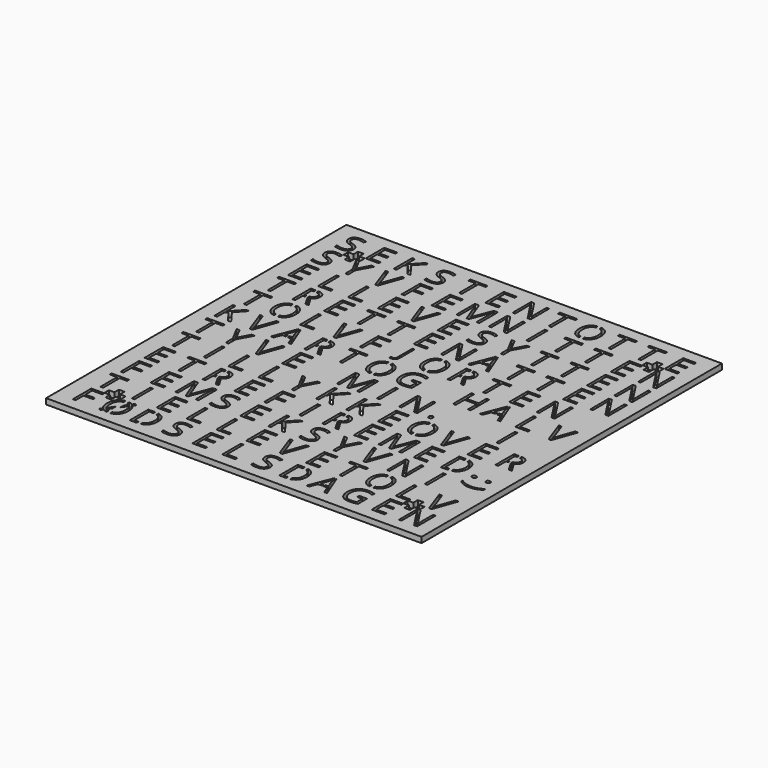
from build123d import *

# Parameters (mm, degrees)
F0_W            = 195
F0_H            = 195
F1_DEPTH        = 3
F2_W            = 3
F2_H            = 3
F3_DEPTH        = 3.001
F5_TEXT_SIZE    = 17.3611111111
F28_DEPTH       = 3.001
F6_TEXT_SIZE    = 17.3611111111
F29_DEPTH       = 3.0010001
F7_TEXT_SIZE    = 17.3611111111
F30_DEPTH       = 3.0010001
F8_TEXT_SIZE    = 17.3611111111
F31_DEPTH       = 3.0010001
F9_TEXT_SIZE    = 17.3611111111
F32_DEPTH       = 3.0010001
F10_TEXT_SIZE   = 17.3611111111
F33_DEPTH       = 3.0010001
F11_TEXT_SIZE   = 17.3611111111
F34_DEPTH       = 3.0010001
F12_TEXT_SIZE   = 17.3611111111
F12_TEXT_SIZE_2 = 13.8888888889
F35_DEPTH       = 3.0010001
F13_TEXT_SIZE   = 17.3611111111
F36_DEPTH       = 3.0010001
F14_TEXT_SIZE   = 17.3611111111
F37_DEPTH       = 3.0010001
F15_TEXT_SIZE   = 17.3611111111
F38_DEPTH       = 3.0010001
F16_TEXT_SIZE   = 17.3611111111
F17_TEXT_SIZE   = 17.3611111111
F18_TEXT_SIZE   = 17.3611111111
F39_DEPTH       = 3.0010001
F19_TEXT_SIZE   = 17.3611111111
F40_DEPTH       = 3.0010001
F20_TEXT_SIZE   = 17.3611111111
F41_DEPTH       = 3.0010001
F21_TEXT_SIZE   = 17.3611111111
F42_DEPTH       = 3.0010001
F24_TEXT_SIZE   = 17.3611111111
F22_TEXT_SIZE   = 17.3611111111
F23_TEXT_SIZE   = 17.3611111111
F23_TEXT_SIZE_2 = 13.8888888889
F43_DEPTH       = 3.0010001
F25_TEXT_SIZE   = 17.3611111111
F44_DEPTH       = 3.0010001
F26_TEXT_SIZE   = 17.3611111111
F45_DEPTH       = 3.0010001
F27_TEXT_SIZE   = 17.3611111111
F46_DEPTH       = 25
F47_DEPTH       = 3
F48_DEPTH       = 3
F49_DEPTH       = 3
F50_DEPTH       = 3


# Not quite as in the source:
# - Text() gives the source's letters only with a copy of the font that has no kerning and outlines rounded to 1/6400 em; it was checked with that copy


with BuildPart() as f1:
    # F0 (on Top) → F1 (new body)
    with BuildSketch(Plane.XY):
        Rectangle(F0_W, F0_H)
    extrude(amount=F1_DEPTH)

    # F2 (on face) → F3 (cut, through all)
    with BuildSketch(Plane.XY.offset(3)):
        with Locations((-83, 80)):
            Rectangle(F2_W, F2_H)
        with Locations((-80, 80)):
            Rectangle(F2_W, F2_H)
        with Locations((-80, 83)):
            Rectangle(F2_W, F2_H)
        with Locations((-77, 80)):
            Rectangle(F2_W, F2_H)
        with Locations((-80, 77)):
            Rectangle(F2_W, F2_H)
        with Locations((77, 80)):
            Rectangle(F2_W, F2_H)
        with Locations((80, 83)):
            Rectangle(F2_W, F2_H)
        with Locations((80, 77)):
            Rectangle(F2_W, F2_H)
        with Locations((83, 80)):
            Rectangle(F2_W, F2_H)
        with Locations((80, 80)):
            Rectangle(F2_W, F2_H)
        with Locations((80, -80)):
            Rectangle(F2_W, F2_H)
        with Locations((-80, -83)):
            Rectangle(F2_W, F2_H)
        with Locations((80, -83)):
            Rectangle(F2_W, F2_H)
        with Locations((77, -80)):
            Rectangle(F2_W, F2_H)
        with Locations((-80, -80)):
            Rectangle(F2_W, F2_H)
        with Locations((-80, -77)):
            Rectangle(F2_W, F2_H)
        with Locations((-83, -80)):
            Rectangle(F2_W, F2_H)
        with Locations((-77, -80)):
            Rectangle(F2_W, F2_H)
        with Locations((83, -80)):
            Rectangle(F2_W, F2_H)
        with Locations((80, -77)):
            Rectangle(F2_W, F2_H)
    extrude(amount=-F3_DEPTH, mode=Mode.SUBTRACT)

    # F5 (on face) → F28 (cut, through all)
    with BuildSketch(Plane.XY.offset(3)):
        with BuildLine():
            add(Edge.make_bspline(
                [(41, 94.2741594654), (42.9624487495, 94.006635936), (44.1680230035, 92.6440972222)],
                knots=[0.1963419657, 0.1963419657, 0.1963419657, 1, 1, 1], degree=2))
            Line((41, 94.2741594654), (41, 92.9625807227))
            add(Edge.make_bspline(
                [(43.0938042535, 91.7584092882), (42.3205692357, 92.7129338633), (41, 92.9625807227)],
                knots=[0, 0, 0, 0.738459474, 0.738459474, 0.738459474], degree=2))
            add(Edge.make_bspline(
                [(44.1408962674, 87.9647352431), (44.1408962674, 90.4658203125), (43.0938042535, 91.7584092882)],
                knots=[0, 0, 0, 1, 1, 1], degree=2))
            add(Edge.make_bspline(
                [(43.0897352431, 84.1398654514), (44.1408962674, 85.4365234375), (44.1408962674, 87.9647352431)],
                knots=[0, 0, 0, 1, 1, 1], degree=2))
            add(Edge.make_bspline(
                [(41, 82.9342437314), (42.3170989399, 83.1867811858), (43.0897352431, 84.1398654514)],
                knots=[0.2649686534, 0.2649686534, 0.2649686534, 1, 1, 1], degree=2))
            Line((41, 82.9342437314), (41, 81.6467767811))
            add(Edge.make_bspline(
                [(44.1625976562, 83.2840169271), (42.9570173112, 81.9187786444), (41, 81.6467767811)],
                knots=[0, 0, 0, 0.8007660152, 0.8007660152, 0.8007660152], degree=2))
            add(Edge.make_bspline(
                [(45.6681315104, 87.9647352431), (45.6681315104, 84.9889322917), (44.1625976562, 83.2840169271)],
                knots=[0, 0, 0, 1, 1, 1], degree=2))
            add(Edge.make_bspline(
                [(44.1680230035, 92.6440972222), (45.6681315104, 90.9486762153), (45.6681315104, 87.9647352431)],
                knots=[0, 0, 0, 1, 1, 1], degree=2))
        make_face()
        with BuildLine():
            Line((39, 92.9644818436), (39, 94.2796444382))
            add(Edge.make_bspline(
                [(35.758734809, 92.6739366319), (36.9678295875, 94.0237260755), (39, 94.2796444382)],
                knots=[0, 0, 0, 0.8104012711, 0.8104012711, 0.8104012711], degree=2))
            add(Edge.make_bspline(
                [(34.2667643229, 87.9810112847), (34.2667643229, 91.0083550347), (35.758734809, 92.6739366319)],
                knots=[0, 0, 0, 1, 1, 1], degree=2))
            add(Edge.make_bspline(
                [(35.7546657986, 83.2541775174), (34.2667643229, 84.9292534722), (34.2667643229, 87.9810112847)],
                knots=[0, 0, 0, 1, 1, 1], degree=2))
            add(Edge.make_bspline(
                [(39, 81.6376356301), (36.9644286676, 81.8922293467), (35.7546657986, 83.2541775174)],
                knots=[0.186933484, 0.186933484, 0.186933484, 1, 1, 1], degree=2))
            Line((39, 81.6376356301), (39, 82.9280543594))
            add(Edge.make_bspline(
                [(36.8641493056, 84.1452907986), (37.6631428834, 83.1755893641), (39, 82.9280543594)],
                knots=[0, 0, 0, 0.7447307017, 0.7447307017, 0.7447307017], degree=2))
            add(Edge.make_bspline(
                [(35.7912868924, 87.9647352431), (35.7912868924, 85.4473741319), (36.8641493056, 84.1452907986)],
                knots=[0, 0, 0, 1, 1, 1], degree=2))
            add(Edge.make_bspline(
                [(36.8641493056, 91.7489149306), (35.7912868924, 90.4468315972), (35.7912868924, 87.9647352431)],
                knots=[0, 0, 0, 1, 1, 1], degree=2))
            add(Edge.make_bspline(
                [(39, 92.9644818436), (37.6604615605, 92.7153621678), (36.8641493056, 91.7489149306)],
                knots=[0.2577685218, 0.2577685218, 0.2577685218, 1, 1, 1], degree=2))
        make_face()
        with Locations((50.7157118056, 81.75)):
            Text('T', F5_TEXT_SIZE, font='Open Sans', text_align=(TextAlign.LEFT, TextAlign.BOTTOM))
        with Locations((18.7157118056, 81.75)):
            Text('T', F5_TEXT_SIZE, font='Open Sans', text_align=(TextAlign.LEFT, TextAlign.BOTTOM))
        with Locations((1.7445746528, 81.75)):
            Text('N', F5_TEXT_SIZE, font='Open Sans', text_align=(TextAlign.LEFT, TextAlign.BOTTOM))
        with Locations((-12.8692491319, 81.75)):
            Text('E', F5_TEXT_SIZE, font='Open Sans', text_align=(TextAlign.LEFT, TextAlign.BOTTOM))
        with Locations((-29.2842881944, 81.75)):
            Text('T', F5_TEXT_SIZE, font='Open Sans', text_align=(TextAlign.LEFT, TextAlign.BOTTOM))
        with Locations((-44.9112955729, 81.75)):
            Text('S', F5_TEXT_SIZE, font='Open Sans', text_align=(TextAlign.LEFT, TextAlign.BOTTOM))
        with Locations((-61.8905707465, 81.75)):
            Text('K', F5_TEXT_SIZE, font='Open Sans', text_align=(TextAlign.LEFT, TextAlign.BOTTOM))
        with Locations((-76.8692491319, 81.75)):
            Text('E', F5_TEXT_SIZE, font='Open Sans', text_align=(TextAlign.LEFT, TextAlign.BOTTOM))
        with Locations((-92.9112955729, 81.75)):
            Text('S', F5_TEXT_SIZE, font='Open Sans', text_align=(TextAlign.LEFT, TextAlign.BOTTOM))
    extrude(amount=-F28_DEPTH, mode=Mode.SUBTRACT)

    # F6 (on face) → F29 (cut, through all)
    with BuildSketch(Plane.XY.offset(3)):
        with Locations((66.7157118056, 81.75)):
            Text('T', F6_TEXT_SIZE, font='Open Sans', text_align=(TextAlign.LEFT, TextAlign.BOTTOM))
        with Locations((83.1307508681, 81.75)):
            Text('E', F6_TEXT_SIZE, font='Open Sans', text_align=(TextAlign.LEFT, TextAlign.BOTTOM))
    extrude(amount=-F29_DEPTH, mode=Mode.SUBTRACT)

    # F7 (on face) → F30 (cut, through all)
    with BuildSketch(Plane.XY.offset(3)):
        with Locations((-92.9112955729, 65.75)):
            Text('S', F7_TEXT_SIZE, font='Open Sans', text_align=(TextAlign.LEFT, TextAlign.BOTTOM))
        with Locations((-77.4239908854, 65.75)):
            Text('Y', F7_TEXT_SIZE, font='Open Sans', text_align=(TextAlign.LEFT, TextAlign.BOTTOM))
        with Locations((-61.7291666667, 65.75)):
            Text('V', F7_TEXT_SIZE, font='Open Sans', text_align=(TextAlign.LEFT, TextAlign.BOTTOM))
        with Locations((-44.8692491319, 65.75)):
            Text('F', F7_TEXT_SIZE, font='Open Sans', text_align=(TextAlign.LEFT, TextAlign.BOTTOM))
        with Locations((-28.8692491319, 65.75)):
            Text('E', F7_TEXT_SIZE, font='Open Sans', text_align=(TextAlign.LEFT, TextAlign.BOTTOM))
        with Locations((-15.5520833333, 65.75)):
            Text('M', F7_TEXT_SIZE, font='Open Sans', text_align=(TextAlign.LEFT, TextAlign.BOTTOM))
        with Locations((1.7445746528, 65.75)):
            Text('N', F7_TEXT_SIZE, font='Open Sans', text_align=(TextAlign.LEFT, TextAlign.BOTTOM))
        with Locations((21.8651258681, 65.75)):
            Text('I', F7_TEXT_SIZE, font='Open Sans', text_align=(TextAlign.LEFT, TextAlign.BOTTOM))
        with Locations((34.7157118056, 65.75)):
            Text('T', F7_TEXT_SIZE, font='Open Sans', text_align=(TextAlign.LEFT, TextAlign.BOTTOM))
        with Locations((50.7157118056, 65.75)):
            Text('T', F7_TEXT_SIZE, font='Open Sans', text_align=(TextAlign.LEFT, TextAlign.BOTTOM))
        with Locations((67.1307508681, 65.75)):
            Text('E', F7_TEXT_SIZE, font='Open Sans', text_align=(TextAlign.LEFT, TextAlign.BOTTOM))
        with Locations((81.7445746528, 65.75)):
            Text('N', F7_TEXT_SIZE, font='Open Sans', text_align=(TextAlign.LEFT, TextAlign.BOTTOM))
    extrude(amount=-F30_DEPTH, mode=Mode.SUBTRACT)

    # F8 (on face) → F31 (cut, through all)
    with BuildSketch(Plane.XY.offset(3)):
        with Locations((-92.8692491319, 49.75)):
            Text('E', F8_TEXT_SIZE, font='Open Sans', text_align=(TextAlign.LEFT, TextAlign.BOTTOM))
        with Locations((-76.8692491319, 49.75)):
            Text('L', F8_TEXT_SIZE, font='Open Sans', text_align=(TextAlign.LEFT, TextAlign.BOTTOM))
        with Locations((-60.8692491319, 49.75)):
            Text('L', F8_TEXT_SIZE, font='Open Sans', text_align=(TextAlign.LEFT, TextAlign.BOTTOM))
        with Locations((-44.8692491319, 49.75)):
            Text('E', F8_TEXT_SIZE, font='Open Sans', text_align=(TextAlign.LEFT, TextAlign.BOTTOM))
        with Locations((-29.7291666667, 49.75)):
            Text('V', F8_TEXT_SIZE, font='Open Sans', text_align=(TextAlign.LEFT, TextAlign.BOTTOM))
        with Locations((-12.8692491319, 49.75)):
            Text('E', F8_TEXT_SIZE, font='Open Sans', text_align=(TextAlign.LEFT, TextAlign.BOTTOM))
    extrude(amount=-F31_DEPTH, mode=Mode.SUBTRACT)

    # F9 (on face) → F32 (cut, through all)
    with BuildSketch(Plane.XY.offset(3)):
        with Locations((3.0887044271, 49.75)):
            Text('S', F9_TEXT_SIZE, font='Open Sans', text_align=(TextAlign.LEFT, TextAlign.BOTTOM))
        with Locations((18.5760091146, 49.75)):
            Text('Y', F9_TEXT_SIZE, font='Open Sans', text_align=(TextAlign.LEFT, TextAlign.BOTTOM))
        with Locations((34.7157118056, 49.75)):
            Text('T', F9_TEXT_SIZE, font='Open Sans', text_align=(TextAlign.LEFT, TextAlign.BOTTOM))
        with Locations((50.7157118056, 49.75)):
            Text('T', F9_TEXT_SIZE, font='Open Sans', text_align=(TextAlign.LEFT, TextAlign.BOTTOM))
        with Locations((67.1307508681, 49.75)):
            Text('E', F9_TEXT_SIZE, font='Open Sans', text_align=(TextAlign.LEFT, TextAlign.BOTTOM))
        with Locations((81.7445746528, 49.75)):
            Text('N', F9_TEXT_SIZE, font='Open Sans', text_align=(TextAlign.LEFT, TextAlign.BOTTOM))
    extrude(amount=-F32_DEPTH, mode=Mode.SUBTRACT)

    # F10 (on face) → F33 (cut, through all)
    with BuildSketch(Plane.XY.offset(3)):
        with Locations((-93.2842881944, 33.75)):
            Text('T', F10_TEXT_SIZE, font='Open Sans', text_align=(TextAlign.LEFT, TextAlign.BOTTOM))
        Polygon((-74.63671875, 38.9040798611), (-73.5, 38.9040798611), (-73.5, 40.1410590278), (-74.63671875, 40.1410590278), (-74.63671875, 44.8800998264), (-73.5, 44.8800998264), (-73.5, 46.1442057292), (-76.0771484375, 46.1442057292), (-76.0771484375, 33.75), (-74.63671875, 33.75), align=None)
        with BuildLine():
            Line((-72, 40.1732229439), (-72, 38.8201979104))
            Line((-72, 38.8201979104), (-69.0486111111, 33.75))
            Line((-69.0486111111, 33.75), (-67.3450520833, 33.75))
            Line((-67.3450520833, 33.75), (-70.7114800347, 39.3191189236))
            add(Edge.make_bspline(
                [(-68.2185329861, 42.6421440972), (-68.2185329861, 40.1844618056), (-70.7114800347, 39.3191189236)],
                knots=[0, 0, 0, 1, 1, 1], degree=2))
            add(Edge.make_bspline(
                [(-69.307671441, 45.2707248264), (-68.2185329861, 44.3972439236), (-68.2185329861, 42.6421440972)],
                knots=[0, 0, 0, 1, 1, 1], degree=2))
            add(Edge.make_bspline(
                [(-72, 46.1232467952), (-70.2280998357, 46.0089015216), (-69.307671441, 45.2707248264)],
                knots=[0.1549023077, 0.1549023077, 0.1549023077, 1, 1, 1], degree=2))
            Line((-72, 46.1232467952), (-72, 44.8446421518))
            add(Edge.make_bspline(
                [(-70.4347873264, 44.3375651042), (-70.9739099068, 44.7414022431), (-72, 44.8446421518)],
                knots=[0, 0, 0, 0.7443526144, 0.7443526144, 0.7443526144], degree=2))
            add(Edge.make_bspline(
                [(-69.7105034722, 42.5661892361), (-69.7105034722, 43.7950303819), (-70.4347873264, 44.3375651042)],
                knots=[0, 0, 0, 1, 1, 1], degree=2))
            add(Edge.make_bspline(
                [(-70.4225802951, 40.7473415799), (-69.7105034722, 41.3536241319), (-69.7105034722, 42.5661892361)],
                knots=[0, 0, 0, 1, 1, 1], degree=2))
            add(Edge.make_bspline(
                [(-72, 40.1732229439), (-70.9706458163, 40.2807029362), (-70.4225802951, 40.7473415799)],
                knots=[0.2303281002, 0.2303281002, 0.2303281002, 1, 1, 1], degree=2))
        make_face()
        with Locations((-60.8692491319, 33.75)):
            Text('E', F10_TEXT_SIZE, font='Open Sans', text_align=(TextAlign.LEFT, TextAlign.BOTTOM))
        with Locations((-45.2842881944, 33.75)):
            Text('T', F10_TEXT_SIZE, font='Open Sans', text_align=(TextAlign.LEFT, TextAlign.BOTTOM))
        with Locations((-29.2842881944, 33.75)):
            Text('T', F10_TEXT_SIZE, font='Open Sans', text_align=(TextAlign.LEFT, TextAlign.BOTTOM))
        with Locations((-12.8692491319, 33.75)):
            Text('E', F10_TEXT_SIZE, font='Open Sans', text_align=(TextAlign.LEFT, TextAlign.BOTTOM))
    extrude(amount=-F33_DEPTH, mode=Mode.SUBTRACT)

    # F11 (on face) → F34 (cut, through all)
    with BuildSketch(Plane.XY.offset(3)):
        with Locations((1.7445746528, 33.75)):
            Text('N', F11_TEXT_SIZE, font='Open Sans', text_align=(TextAlign.LEFT, TextAlign.BOTTOM))
        with BuildLine():
            Line((22.9551373869, 43.0014366443), (22.9551373869, 46.1957465278))
            Line((22.9551373869, 46.1957465278), (22.8430447049, 46.1957465278))
            Line((22.8430447049, 46.1957465278), (17.9439561632, 33.75))
            Line((17.9439561632, 33.75), (19.403374566, 33.75))
            Line((19.403374566, 33.75), (20.9278971354, 37.6915147569))
            Line((20.9278971354, 37.6915147569), (22.9551373869, 37.6915147569))
            Line((22.9551373869, 37.6915147569), (22.9551373869, 38.9881727431))
            Line((22.9551373869, 38.9881727431), (21.4378797743, 38.9881727431))
            Line((21.4378797743, 38.9881727431), (22.8945855035, 42.8293185764))
            add(Edge.make_bspline(
                [(22.9551373869, 43.0014366443), (22.9254956152, 42.9160117803), (22.8945855035, 42.8293185764)],
                knots=[0.9109788783, 0.9109788783, 0.9109788783, 1, 1, 1], degree=2))
        make_face()
        with BuildLine():
            Line((24.055609809, 46.1957465278), (23.9551373869, 46.1957465278))
            Line((23.9551373869, 46.1957465278), (23.9551373869, 42.9592905556))
            add(Edge.make_bspline(
                [(24.0040690104, 42.8293185764), (23.9796652801, 42.8930525905), (23.9551373869, 42.9592905556)],
                knots=[0, 0, 0, 0.0873416616, 0.0873416616, 0.0873416616], degree=2))
            Line((24.0040690104, 42.8293185764), (25.4472113715, 38.9881727431))
            Line((25.4472113715, 38.9881727431), (23.9551373869, 38.9881727431))
            Line((23.9551373869, 38.9881727431), (23.9551373869, 37.6915147569))
            Line((23.9551373869, 37.6915147569), (25.8948025174, 37.6915147569))
            Line((25.8948025174, 37.6915147569), (27.4383138021, 33.75))
            Line((27.4383138021, 33.75), (28.9302842882, 33.75))
            Line((28.9302842882, 33.75), (24.055609809, 46.1957465278))
        make_face()
        with Locations((34.7157118056, 33.75)):
            Text('T', F11_TEXT_SIZE, font='Open Sans', text_align=(TextAlign.LEFT, TextAlign.BOTTOM))
        with Locations((50.7157118056, 33.75)):
            Text('T', F11_TEXT_SIZE, font='Open Sans', text_align=(TextAlign.LEFT, TextAlign.BOTTOM))
        with Locations((67.1307508681, 33.75)):
            Text('E', F11_TEXT_SIZE, font='Open Sans', text_align=(TextAlign.LEFT, TextAlign.BOTTOM))
        with Locations((81.7445746528, 33.75)):
            Text('N', F11_TEXT_SIZE, font='Open Sans', text_align=(TextAlign.LEFT, TextAlign.BOTTOM))
    extrude(amount=-F34_DEPTH, mode=Mode.SUBTRACT)

    # F12 (on face) → F35 (cut, through all)
    with BuildSketch(Plane.XY.offset(3)):
        with Locations((-93.2842881944, 17.75)):
            Text('T', F12_TEXT_SIZE, font='Open Sans', text_align=(TextAlign.LEFT, TextAlign.BOTTOM))
        with BuildLine():
            Line((-73, 28.9644818436), (-73, 30.2796444382))
            add(Edge.make_bspline(
                [(-76.241265191, 28.6739366319), (-75.0321704125, 30.0237260755), (-73, 30.2796444382)],
                knots=[0, 0, 0, 0.8104012711, 0.8104012711, 0.8104012711], degree=2))
            add(Edge.make_bspline(
                [(-77.7332356771, 23.9810112847), (-77.7332356771, 27.0083550347), (-76.241265191, 28.6739366319)],
                knots=[0, 0, 0, 1, 1, 1], degree=2))
            add(Edge.make_bspline(
                [(-76.2453342014, 19.2541775174), (-77.7332356771, 20.9292534722), (-77.7332356771, 23.9810112847)],
                knots=[0, 0, 0, 1, 1, 1], degree=2))
            add(Edge.make_bspline(
                [(-73, 17.6376356301), (-75.0355713324, 17.8922293467), (-76.2453342014, 19.2541775174)],
                knots=[0.186933484, 0.186933484, 0.186933484, 1, 1, 1], degree=2))
            Line((-73, 17.6376356301), (-73, 18.9280543594))
            add(Edge.make_bspline(
                [(-75.1358506944, 20.1452907986), (-74.3368571166, 19.1755893641), (-73, 18.9280543594)],
                knots=[0, 0, 0, 0.7447307017, 0.7447307017, 0.7447307017], degree=2))
            add(Edge.make_bspline(
                [(-76.2087131076, 23.9647352431), (-76.2087131076, 21.4473741319), (-75.1358506944, 20.1452907986)],
                knots=[0, 0, 0, 1, 1, 1], degree=2))
            add(Edge.make_bspline(
                [(-75.1358506944, 27.7489149306), (-76.2087131076, 26.4468315972), (-76.2087131076, 23.9647352431)],
                knots=[0, 0, 0, 1, 1, 1], degree=2))
            add(Edge.make_bspline(
                [(-73, 28.9644818436), (-74.3395384395, 28.7153621678), (-75.1358506944, 27.7489149306)],
                knots=[0.2577685218, 0.2577685218, 0.2577685218, 1, 1, 1], degree=2))
        make_face()
        with BuildLine():
            add(Edge.make_bspline(
                [(-71, 30.2741594654), (-69.0375512505, 30.006635936), (-67.8319769965, 28.6440972222)],
                knots=[0.1963419657, 0.1963419657, 0.1963419657, 1, 1, 1], degree=2))
            Line((-71, 30.2741594654), (-71, 28.9625807227))
            add(Edge.make_bspline(
                [(-68.9061957465, 27.7584092882), (-69.6794307643, 28.7129338633), (-71, 28.9625807227)],
                knots=[0, 0, 0, 0.738459474, 0.738459474, 0.738459474], degree=2))
            add(Edge.make_bspline(
                [(-67.8591037326, 23.9647352431), (-67.8591037326, 26.4658203125), (-68.9061957465, 27.7584092882)],
                knots=[0, 0, 0, 1, 1, 1], degree=2))
            add(Edge.make_bspline(
                [(-68.9102647569, 20.1398654514), (-67.8591037326, 21.4365234375), (-67.8591037326, 23.9647352431)],
                knots=[0, 0, 0, 1, 1, 1], degree=2))
            add(Edge.make_bspline(
                [(-71, 18.9342437314), (-69.6829010601, 19.1867811858), (-68.9102647569, 20.1398654514)],
                knots=[0.2649686534, 0.2649686534, 0.2649686534, 1, 1, 1], degree=2))
            Line((-71, 18.9342437314), (-71, 17.6467767811))
            add(Edge.make_bspline(
                [(-67.8374023437, 19.2840169271), (-69.0429826888, 17.9187786444), (-71, 17.6467767811)],
                knots=[0, 0, 0, 0.8007660152, 0.8007660152, 0.8007660152], degree=2))
            add(Edge.make_bspline(
                [(-66.3318684896, 23.9647352431), (-66.3318684896, 20.9889322917), (-67.8374023437, 19.2840169271)],
                knots=[0, 0, 0, 1, 1, 1], degree=2))
            add(Edge.make_bspline(
                [(-67.8319769965, 28.6440972222), (-66.3318684896, 26.9486762153), (-66.3318684896, 23.9647352431)],
                knots=[0, 0, 0, 1, 1, 1], degree=2))
        make_face()
        with Locations((-60.8692491319, 17.75)):
            Text('L', F12_TEXT_SIZE, font='Open Sans', text_align=(TextAlign.LEFT, TextAlign.BOTTOM))
        with Locations((-45.7291666667, 17.75)):
            Text('V', F12_TEXT_SIZE, font='Open Sans', text_align=(TextAlign.LEFT, TextAlign.BOTTOM))
        with Locations((-28.8692491319, 17.75)):
            Text('F', F12_TEXT_SIZE, font='Open Sans', text_align=(TextAlign.LEFT, TextAlign.BOTTOM))
        with Locations((-10.2135416667, 20.25)):
            Text('J', F12_TEXT_SIZE_2, font='Open Sans', text_align=(TextAlign.LEFT, TextAlign.BOTTOM))
    extrude(amount=-F35_DEPTH, mode=Mode.SUBTRACT)

    # F13 (on face) → F36 (cut, through all)
    with BuildSketch(Plane.XY.offset(3)):
        with BuildLine():
            Line((7, 28.9644818436), (7, 30.2796444382))
            add(Edge.make_bspline(
                [(3.758734809, 28.6739366319), (4.9678295875, 30.0237260755), (7, 30.2796444382)],
                knots=[0, 0, 0, 0.8104012711, 0.8104012711, 0.8104012711], degree=2))
            add(Edge.make_bspline(
                [(2.2667643229, 23.9810112847), (2.2667643229, 27.0083550347), (3.758734809, 28.6739366319)],
                knots=[0, 0, 0, 1, 1, 1], degree=2))
            add(Edge.make_bspline(
                [(3.7546657986, 19.2541775174), (2.2667643229, 20.9292534722), (2.2667643229, 23.9810112847)],
                knots=[0, 0, 0, 1, 1, 1], degree=2))
            add(Edge.make_bspline(
                [(7, 17.6376356301), (4.9644286676, 17.8922293467), (3.7546657986, 19.2541775174)],
                knots=[0.186933484, 0.186933484, 0.186933484, 1, 1, 1], degree=2))
            Line((7, 17.6376356301), (7, 18.9280543594))
            add(Edge.make_bspline(
                [(4.8641493056, 20.1452907986), (5.6631428834, 19.1755893641), (7, 18.9280543594)],
                knots=[0, 0, 0, 0.7447307017, 0.7447307017, 0.7447307017], degree=2))
            add(Edge.make_bspline(
                [(3.7912868924, 23.9647352431), (3.7912868924, 21.4473741319), (4.8641493056, 20.1452907986)],
                knots=[0, 0, 0, 1, 1, 1], degree=2))
            add(Edge.make_bspline(
                [(4.8641493056, 27.7489149306), (3.7912868924, 26.4468315972), (3.7912868924, 23.9647352431)],
                knots=[0, 0, 0, 1, 1, 1], degree=2))
            add(Edge.make_bspline(
                [(7, 28.9644818436), (5.6604615605, 28.7153621678), (4.8641493056, 27.7489149306)],
                knots=[0.2577685218, 0.2577685218, 0.2577685218, 1, 1, 1], degree=2))
        make_face()
        with BuildLine():
            add(Edge.make_bspline(
                [(9, 30.2741594654), (10.9624487495, 30.006635936), (12.1680230035, 28.6440972222)],
                knots=[0.1963419657, 0.1963419657, 0.1963419657, 1, 1, 1], degree=2))
            Line((9, 30.2741594654), (9, 28.9625807227))
            add(Edge.make_bspline(
                [(11.0938042535, 27.7584092882), (10.3205692357, 28.7129338633), (9, 28.9625807227)],
                knots=[0, 0, 0, 0.738459474, 0.738459474, 0.738459474], degree=2))
            add(Edge.make_bspline(
                [(12.1408962674, 23.9647352431), (12.1408962674, 26.4658203125), (11.0938042535, 27.7584092882)],
                knots=[0, 0, 0, 1, 1, 1], degree=2))
            add(Edge.make_bspline(
                [(11.0897352431, 20.1398654514), (12.1408962674, 21.4365234375), (12.1408962674, 23.9647352431)],
                knots=[0, 0, 0, 1, 1, 1], degree=2))
            add(Edge.make_bspline(
                [(9, 18.9342437314), (10.3170989399, 19.1867811858), (11.0897352431, 20.1398654514)],
                knots=[0.2649686534, 0.2649686534, 0.2649686534, 1, 1, 1], degree=2))
            Line((9, 18.9342437314), (9, 17.6467767811))
            add(Edge.make_bspline(
                [(12.1625976562, 19.2840169271), (10.9570173112, 17.9187786444), (9, 17.6467767811)],
                knots=[0, 0, 0, 0.8007660152, 0.8007660152, 0.8007660152], degree=2))
            add(Edge.make_bspline(
                [(13.6681315104, 23.9647352431), (13.6681315104, 20.9889322917), (12.1625976562, 19.2840169271)],
                knots=[0, 0, 0, 1, 1, 1], degree=2))
            add(Edge.make_bspline(
                [(12.1680230035, 28.6440972222), (13.6681315104, 26.9486762153), (13.6681315104, 23.9647352431)],
                knots=[0, 0, 0, 1, 1, 1], degree=2))
        make_face()
        Polygon((21.36328125, 22.9040798611), (22.5, 22.9040798611), (22.5, 24.1410590278), (21.36328125, 24.1410590278), (21.36328125, 28.8800998264), (22.5, 28.8800998264), (22.5, 30.1442057292), (19.9228515625, 30.1442057292), (19.9228515625, 17.75), (21.36328125, 17.75), align=None)
        with BuildLine():
            Line((24, 24.1732229439), (24, 22.8201979104))
            Line((24, 22.8201979104), (26.9513888889, 17.75))
            Line((26.9513888889, 17.75), (28.6549479167, 17.75))
            Line((28.6549479167, 17.75), (25.2885199653, 23.3191189236))
            add(Edge.make_bspline(
                [(27.7814670139, 26.6421440972), (27.7814670139, 24.1844618056), (25.2885199653, 23.3191189236)],
                knots=[0, 0, 0, 1, 1, 1], degree=2))
            add(Edge.make_bspline(
                [(26.692328559, 29.2707248264), (27.7814670139, 28.3972439236), (27.7814670139, 26.6421440972)],
                knots=[0, 0, 0, 1, 1, 1], degree=2))
            add(Edge.make_bspline(
                [(24, 30.1232467952), (25.7719001643, 30.0089015216), (26.692328559, 29.2707248264)],
                knots=[0.1549023077, 0.1549023077, 0.1549023077, 1, 1, 1], degree=2))
            Line((24, 30.1232467952), (24, 28.8446421518))
            add(Edge.make_bspline(
                [(25.5652126736, 28.3375651042), (25.0260900932, 28.7414022431), (24, 28.8446421518)],
                knots=[0, 0, 0, 0.7443526144, 0.7443526144, 0.7443526144], degree=2))
            add(Edge.make_bspline(
                [(26.2894965278, 26.5661892361), (26.2894965278, 27.7950303819), (25.5652126736, 28.3375651042)],
                knots=[0, 0, 0, 1, 1, 1], degree=2))
            add(Edge.make_bspline(
                [(25.5774197049, 24.7473415799), (26.2894965278, 25.3536241319), (26.2894965278, 26.5661892361)],
                knots=[0, 0, 0, 1, 1, 1], degree=2))
            add(Edge.make_bspline(
                [(24, 24.1732229439), (25.0293541837, 24.2807029362), (25.5774197049, 24.7473415799)],
                knots=[0.2303281002, 0.2303281002, 0.2303281002, 1, 1, 1], degree=2))
        make_face()
        with Locations((34.7157118056, 17.75)):
            Text('T', F13_TEXT_SIZE, font='Open Sans', text_align=(TextAlign.LEFT, TextAlign.BOTTOM))
        with Locations((51.1307508681, 17.75)):
            Text('E', F13_TEXT_SIZE, font='Open Sans', text_align=(TextAlign.LEFT, TextAlign.BOTTOM))
        with Locations((65.7445746528, 17.75)):
            Text('N', F13_TEXT_SIZE, font='Open Sans', text_align=(TextAlign.LEFT, TextAlign.BOTTOM))
    extrude(amount=-F36_DEPTH, mode=Mode.SUBTRACT)

    # F14 (on face) → F37 (cut, through all)
    with BuildSketch(Plane.XY.offset(3)):
        with Locations((-93.8905707465, 1.75)):
            Text('K', F14_TEXT_SIZE, font='Open Sans', text_align=(TextAlign.LEFT, TextAlign.BOTTOM))
        with Locations((-77.7291666667, 1.75)):
            Text('V', F14_TEXT_SIZE, font='Open Sans', text_align=(TextAlign.LEFT, TextAlign.BOTTOM))
        Polygon((-57.1255721152, 10.7761655261), (-57.1255721152, 14.1957465278), (-57.1569552951, 14.1957465278), (-62.0560438368, 1.75), (-60.596625434, 1.75), (-59.0721028646, 5.6915147569), (-57.1255721152, 5.6915147569), (-57.1255721152, 6.9881727431), (-58.5621202257, 6.9881727431), align=None)
        with BuildLine():
            Line((-55.944390191, 14.1957465278), (-56.1255721152, 14.1957465278))
            Line((-56.1255721152, 14.1957465278), (-56.1255721152, 11.1830697261))
            add(Edge.make_bspline(
                [(-55.9959309896, 10.8293185764), (-56.0603193727, 10.9974785285), (-56.1255721152, 11.1830697261)],
                knots=[0, 0, 0, 0.2304478987, 0.2304478987, 0.2304478987], degree=2))
            Line((-55.9959309896, 10.8293185764), (-54.5527886285, 6.9881727431))
            Line((-54.5527886285, 6.9881727431), (-56.1255721152, 6.9881727431))
            Line((-56.1255721152, 6.9881727431), (-56.1255721152, 5.6915147569))
            Line((-56.1255721152, 5.6915147569), (-54.1051974826, 5.6915147569))
            Line((-54.1051974826, 5.6915147569), (-52.5616861979, 1.75))
            Line((-52.5616861979, 1.75), (-51.0697157118, 1.75))
            Line((-51.0697157118, 1.75), (-55.944390191, 14.1957465278))
        make_face()
        Polygon((-42.63671875, 6.9040798611), (-41.5, 6.9040798611), (-41.5, 8.1410590278), (-42.63671875, 8.1410590278), (-42.63671875, 12.8800998264), (-41.5, 12.8800998264), (-41.5, 14.1442057292), (-44.0771484375, 14.1442057292), (-44.0771484375, 1.75), (-42.63671875, 1.75), align=None)
        with BuildLine():
            Line((-40, 8.1732229439), (-40, 6.8201979104))
            Line((-40, 6.8201979104), (-37.0486111111, 1.75))
            Line((-37.0486111111, 1.75), (-35.3450520833, 1.75))
            Line((-35.3450520833, 1.75), (-38.7114800347, 7.3191189236))
            add(Edge.make_bspline(
                [(-36.2185329861, 10.6421440972), (-36.2185329861, 8.1844618056), (-38.7114800347, 7.3191189236)],
                knots=[0, 0, 0, 1, 1, 1], degree=2))
            add(Edge.make_bspline(
                [(-37.307671441, 13.2707248264), (-36.2185329861, 12.3972439236), (-36.2185329861, 10.6421440972)],
                knots=[0, 0, 0, 1, 1, 1], degree=2))
            add(Edge.make_bspline(
                [(-40, 14.1232467952), (-38.2280998357, 14.0089015216), (-37.307671441, 13.2707248264)],
                knots=[0.1549023077, 0.1549023077, 0.1549023077, 1, 1, 1], degree=2))
            Line((-40, 14.1232467952), (-40, 12.8446421518))
            add(Edge.make_bspline(
                [(-38.4347873264, 12.3375651042), (-38.9739099068, 12.7414022431), (-40, 12.8446421518)],
                knots=[0, 0, 0, 0.7443526144, 0.7443526144, 0.7443526144], degree=2))
            add(Edge.make_bspline(
                [(-37.7105034722, 10.5661892361), (-37.7105034722, 11.7950303819), (-38.4347873264, 12.3375651042)],
                knots=[0, 0, 0, 1, 1, 1], degree=2))
            add(Edge.make_bspline(
                [(-38.4225802951, 8.7473415799), (-37.7105034722, 9.3536241319), (-37.7105034722, 10.5661892361)],
                knots=[0, 0, 0, 1, 1, 1], degree=2))
            add(Edge.make_bspline(
                [(-40, 8.1732229439), (-38.9706458163, 8.2807029362), (-38.4225802951, 8.7473415799)],
                knots=[0.2303281002, 0.2303281002, 0.2303281002, 1, 1, 1], degree=2))
        make_face()
        with Locations((-29.2842881944, 1.75)):
            Text('T', F14_TEXT_SIZE, font='Open Sans', text_align=(TextAlign.LEFT, TextAlign.BOTTOM))
        with BuildLine():
            Line((-9, 12.9644818436), (-9, 14.2796444382))
            add(Edge.make_bspline(
                [(-12.241265191, 12.6739366319), (-11.0321704125, 14.0237260755), (-9, 14.2796444382)],
                knots=[0, 0, 0, 0.8104012711, 0.8104012711, 0.8104012711], degree=2))
            add(Edge.make_bspline(
                [(-13.7332356771, 7.9810112847), (-13.7332356771, 11.0083550347), (-12.241265191, 12.6739366319)],
                knots=[0, 0, 0, 1, 1, 1], degree=2))
            add(Edge.make_bspline(
                [(-12.2453342014, 3.2541775174), (-13.7332356771, 4.9292534722), (-13.7332356771, 7.9810112847)],
                knots=[0, 0, 0, 1, 1, 1], degree=2))
            add(Edge.make_bspline(
                [(-9, 1.6376356301), (-11.0355713324, 1.8922293467), (-12.2453342014, 3.2541775174)],
                knots=[0.186933484, 0.186933484, 0.186933484, 1, 1, 1], degree=2))
            Line((-9, 1.6376356301), (-9, 2.9280543594))
            add(Edge.make_bspline(
                [(-11.1358506944, 4.1452907986), (-10.3368571166, 3.1755893641), (-9, 2.9280543594)],
                knots=[0, 0, 0, 0.7447307017, 0.7447307017, 0.7447307017], degree=2))
            add(Edge.make_bspline(
                [(-12.2087131076, 7.9647352431), (-12.2087131076, 5.4473741319), (-11.1358506944, 4.1452907986)],
                knots=[0, 0, 0, 1, 1, 1], degree=2))
            add(Edge.make_bspline(
                [(-11.1358506944, 11.7489149306), (-12.2087131076, 10.4468315972), (-12.2087131076, 7.9647352431)],
                knots=[0, 0, 0, 1, 1, 1], degree=2))
            add(Edge.make_bspline(
                [(-9, 12.9644818436), (-10.3395384395, 12.7153621678), (-11.1358506944, 11.7489149306)],
                knots=[0.2577685218, 0.2577685218, 0.2577685218, 1, 1, 1], degree=2))
        make_face()
        with BuildLine():
            add(Edge.make_bspline(
                [(-7, 14.2741594654), (-5.0375512505, 14.006635936), (-3.8319769965, 12.6440972222)],
                knots=[0.1963419657, 0.1963419657, 0.1963419657, 1, 1, 1], degree=2))
            Line((-7, 14.2741594654), (-7, 12.9625807227))
            add(Edge.make_bspline(
                [(-4.9061957465, 11.7584092882), (-5.6794307643, 12.7129338633), (-7, 12.9625807227)],
                knots=[0, 0, 0, 0.738459474, 0.738459474, 0.738459474], degree=2))
            add(Edge.make_bspline(
                [(-3.8591037326, 7.9647352431), (-3.8591037326, 10.4658203125), (-4.9061957465, 11.7584092882)],
                knots=[0, 0, 0, 1, 1, 1], degree=2))
            add(Edge.make_bspline(
                [(-4.9102647569, 4.1398654514), (-3.8591037326, 5.4365234375), (-3.8591037326, 7.9647352431)],
                knots=[0, 0, 0, 1, 1, 1], degree=2))
            add(Edge.make_bspline(
                [(-7, 2.9342437314), (-5.6829010601, 3.1867811858), (-4.9102647569, 4.1398654514)],
                knots=[0.2649686534, 0.2649686534, 0.2649686534, 1, 1, 1], degree=2))
            Line((-7, 2.9342437314), (-7, 1.6467767811))
            add(Edge.make_bspline(
                [(-3.8374023437, 3.2840169271), (-5.0429826888, 1.9187786444), (-7, 1.6467767811)],
                knots=[0, 0, 0, 0.8007660152, 0.8007660152, 0.8007660152], degree=2))
            add(Edge.make_bspline(
                [(-2.3318684896, 7.9647352431), (-2.3318684896, 4.9889322917), (-3.8374023437, 3.2840169271)],
                knots=[0, 0, 0, 1, 1, 1], degree=2))
            add(Edge.make_bspline(
                [(-3.8319769965, 12.6440972222), (-2.3318684896, 10.9486762153), (-2.3318684896, 7.9647352431)],
                knots=[0, 0, 0, 1, 1, 1], degree=2))
        make_face()
    extrude(amount=-F37_DEPTH, mode=Mode.SUBTRACT)

    # F15 (on face) → F38 (cut, through all)
    with BuildSketch(Plane.XY.offset(3)):
        with Locations((1.7527126736, 1.75)):
            Text('G', F15_TEXT_SIZE, font='Open Sans', text_align=(TextAlign.LEFT, TextAlign.BOTTOM))
        with Locations((33.8802083333, 1.75)):
            Text('H', F15_TEXT_SIZE, font='Open Sans', text_align=(TextAlign.LEFT, TextAlign.BOTTOM))
        with BuildLine():
            Line((54.9337379634, 10.940071765), (54.9337379634, 14.1957465278))
            Line((54.9337379634, 14.1957465278), (54.8430447049, 14.1957465278))
            Line((54.8430447049, 14.1957465278), (49.9439561632, 1.75))
            Line((49.9439561632, 1.75), (51.403374566, 1.75))
            Line((51.403374566, 1.75), (52.9278971354, 5.6915147569))
            Line((52.9278971354, 5.6915147569), (54.9337379634, 5.6915147569))
            Line((54.9337379634, 5.6915147569), (54.9337379634, 6.9881727431))
            Line((54.9337379634, 6.9881727431), (53.4378797743, 6.9881727431))
            Line((53.4378797743, 6.9881727431), (54.8945855035, 10.8293185764))
            add(Edge.make_bspline(
                [(54.9337379634, 10.940071765), (54.9144229348, 10.8849563721), (54.8945855035, 10.8293185764)],
                knots=[0.9428681978, 0.9428681978, 0.9428681978, 1, 1, 1], degree=2))
        make_face()
        with BuildLine():
            Line((56.055609809, 14.1957465278), (55.9337379634, 14.1957465278))
            Line((55.9337379634, 14.1957465278), (55.9337379634, 11.017491809))
            add(Edge.make_bspline(
                [(56.0040690104, 10.8293185764), (55.9690314595, 10.9208244134), (55.9337379634, 11.017491809)],
                knots=[0, 0, 0, 0.1254004154, 0.1254004154, 0.1254004154], degree=2))
            Line((56.0040690104, 10.8293185764), (57.4472113715, 6.9881727431))
            Line((57.4472113715, 6.9881727431), (55.9337379634, 6.9881727431))
            Line((55.9337379634, 6.9881727431), (55.9337379634, 5.6915147569))
            Line((55.9337379634, 5.6915147569), (57.8948025174, 5.6915147569))
            Line((57.8948025174, 5.6915147569), (59.4383138021, 1.75))
            Line((59.4383138021, 1.75), (60.9302842882, 1.75))
            Line((60.9302842882, 1.75), (56.055609809, 14.1957465278))
        make_face()
        with Locations((67.1307508681, 1.75)):
            Text('L', F15_TEXT_SIZE, font='Open Sans', text_align=(TextAlign.LEFT, TextAlign.BOTTOM))
        with Locations((82.2708333333, 1.75)):
            Text('V', F15_TEXT_SIZE, font='Open Sans', text_align=(TextAlign.LEFT, TextAlign.BOTTOM))
    extrude(amount=-F38_DEPTH, mode=Mode.SUBTRACT)

    # F16 (on face) + F17 (on face) + F18 (on face) → F39 (cut, through all)
    with BuildSketch(Plane.XY.offset(3)):
        with Locations((-93.2842881944, -14.25)):
            Text('T', F16_TEXT_SIZE, font='Open Sans', text_align=(TextAlign.LEFT, TextAlign.BOTTOM))
        with Locations((-77.4239908854, -14.25)):
            Text('Y', F16_TEXT_SIZE, font='Open Sans', text_align=(TextAlign.LEFT, TextAlign.BOTTOM))
        with Locations((-61.7291666667, -14.25)):
            Text('V', F16_TEXT_SIZE, font='Open Sans', text_align=(TextAlign.LEFT, TextAlign.BOTTOM))
        with Locations((-15.5520833333, -14.25)):
            Text('M', F16_TEXT_SIZE, font='Open Sans', text_align=(TextAlign.LEFT, TextAlign.BOTTOM))
        with Locations((-44.8692491319, -14.25)):
            Text('E', F16_TEXT_SIZE, font='Open Sans', text_align=(TextAlign.LEFT, TextAlign.BOTTOM))
    with BuildSketch(Plane.XY.offset(3)):
        with Locations((5.8651258681, -14.25)):
            Text('I', F17_TEXT_SIZE, font='Open Sans', text_align=(TextAlign.LEFT, TextAlign.BOTTOM))
        with Locations((17.7445746528, -14.25)):
            Text('N', F17_TEXT_SIZE, font='Open Sans', text_align=(TextAlign.LEFT, TextAlign.BOTTOM))
        with Locations((33.5, -14.25)):
            Text('.', F17_TEXT_SIZE, font='Open Sans', text_align=(TextAlign.LEFT, TextAlign.BOTTOM))
        with Locations((69.8651258681, -14.25)):
            Text('I', F17_TEXT_SIZE, font='Open Sans', text_align=(TextAlign.LEFT, TextAlign.BOTTOM))
    with BuildSketch(Plane.XY.offset(3)):
        with Locations((-93.2842881944, -30.25)):
            Text('T', F18_TEXT_SIZE, font='Open Sans', text_align=(TextAlign.LEFT, TextAlign.BOTTOM))
        with Locations((-74.1348741319, -30.25)):
            Text('I', F18_TEXT_SIZE, font='Open Sans', text_align=(TextAlign.LEFT, TextAlign.BOTTOM))
        with Locations((-44.8692491319, -30.25)):
            Text('L', F18_TEXT_SIZE, font='Open Sans', text_align=(TextAlign.LEFT, TextAlign.BOTTOM))
        with Locations((-60.8692491319, -30.25)):
            Text('L', F18_TEXT_SIZE, font='Open Sans', text_align=(TextAlign.LEFT, TextAlign.BOTTOM))
        with Locations((-29.4239908854, -30.25)):
            Text('Y', F18_TEXT_SIZE, font='Open Sans', text_align=(TextAlign.LEFT, TextAlign.BOTTOM))
        with Locations((-13.8905707465, -30.25)):
            Text('K', F18_TEXT_SIZE, font='Open Sans', text_align=(TextAlign.LEFT, TextAlign.BOTTOM))
    extrude(amount=-F39_DEPTH, mode=Mode.SUBTRACT)

    # F19 (on face) → F40 (cut, through all)
    with BuildSketch(Plane.XY.offset(3)):
        with Locations((2.1094292535, -30.25)):
            Text('K', F19_TEXT_SIZE, font='Open Sans', text_align=(TextAlign.LEFT, TextAlign.BOTTOM))
        with Locations((19.1307508681, -30.25)):
            Text('E', F19_TEXT_SIZE, font='Open Sans', text_align=(TextAlign.LEFT, TextAlign.BOTTOM))
        with BuildLine():
            Line((39, -19.0355181564), (39, -17.7203555618))
            add(Edge.make_bspline(
                [(35.758734809, -19.3260633681), (36.9678295875, -17.9762739245), (39, -17.7203555618)],
                knots=[0, 0, 0, 0.8104012711, 0.8104012711, 0.8104012711], degree=2))
            add(Edge.make_bspline(
                [(34.2667643229, -24.0189887153), (34.2667643229, -20.9916449653), (35.758734809, -19.3260633681)],
                knots=[0, 0, 0, 1, 1, 1], degree=2))
            add(Edge.make_bspline(
                [(35.7546657986, -28.7458224826), (34.2667643229, -27.0707465278), (34.2667643229, -24.0189887153)],
                knots=[0, 0, 0, 1, 1, 1], degree=2))
            add(Edge.make_bspline(
                [(39, -30.3623643699), (36.9644286676, -30.1077706533), (35.7546657986, -28.7458224826)],
                knots=[0.186933484, 0.186933484, 0.186933484, 1, 1, 1], degree=2))
            Line((39, -30.3623643699), (39, -29.0719456406))
            add(Edge.make_bspline(
                [(36.8641493056, -27.8547092014), (37.6631428834, -28.8244106359), (39, -29.0719456406)],
                knots=[0, 0, 0, 0.7447307017, 0.7447307017, 0.7447307017], degree=2))
            add(Edge.make_bspline(
                [(35.7912868924, -24.0352647569), (35.7912868924, -26.5526258681), (36.8641493056, -27.8547092014)],
                knots=[0, 0, 0, 1, 1, 1], degree=2))
            add(Edge.make_bspline(
                [(36.8641493056, -20.2510850694), (35.7912868924, -21.5531684028), (35.7912868924, -24.0352647569)],
                knots=[0, 0, 0, 1, 1, 1], degree=2))
            add(Edge.make_bspline(
                [(39, -19.0355181564), (37.6604615605, -19.2846378322), (36.8641493056, -20.2510850694)],
                knots=[0.2577685218, 0.2577685218, 0.2577685218, 1, 1, 1], degree=2))
        make_face()
        with BuildLine():
            add(Edge.make_bspline(
                [(41, -17.7258405346), (42.9624487495, -17.993364064), (44.1680230035, -19.3559027778)],
                knots=[0.1963419657, 0.1963419657, 0.1963419657, 1, 1, 1], degree=2))
            Line((41, -17.7258405346), (41, -19.0374192773))
            add(Edge.make_bspline(
                [(43.0938042535, -20.2415907118), (42.3205692357, -19.2870661367), (41, -19.0374192773)],
                knots=[0, 0, 0, 0.738459474, 0.738459474, 0.738459474], degree=2))
            add(Edge.make_bspline(
                [(44.1408962674, -24.0352647569), (44.1408962674, -21.5341796875), (43.0938042535, -20.2415907118)],
                knots=[0, 0, 0, 1, 1, 1], degree=2))
            add(Edge.make_bspline(
                [(43.0897352431, -27.8601345486), (44.1408962674, -26.5634765625), (44.1408962674, -24.0352647569)],
                knots=[0, 0, 0, 1, 1, 1], degree=2))
            add(Edge.make_bspline(
                [(41, -29.0657562686), (42.3170989399, -28.8132188142), (43.0897352431, -27.8601345486)],
                knots=[0.2649686534, 0.2649686534, 0.2649686534, 1, 1, 1], degree=2))
            Line((41, -29.0657562686), (41, -30.3532232189))
            add(Edge.make_bspline(
                [(44.1625976563, -28.7159830729), (42.9570173112, -30.0812213556), (41, -30.3532232189)],
                knots=[0, 0, 0, 0.8007660152, 0.8007660152, 0.8007660152], degree=2))
            add(Edge.make_bspline(
                [(45.6681315104, -24.0352647569), (45.6681315104, -27.0110677083), (44.1625976563, -28.7159830729)],
                knots=[0, 0, 0, 1, 1, 1], degree=2))
            add(Edge.make_bspline(
                [(44.1680230035, -19.3559027778), (45.6681315104, -21.0513237847), (45.6681315104, -24.0352647569)],
                knots=[0, 0, 0, 1, 1, 1], degree=2))
        make_face()
        with Locations((50.2708333333, -30.25)):
            Text('V', F19_TEXT_SIZE, font='Open Sans', text_align=(TextAlign.LEFT, TextAlign.BOTTOM))
        with Locations((67.1307508681, -30.25)):
            Text('E', F19_TEXT_SIZE, font='Open Sans', text_align=(TextAlign.LEFT, TextAlign.BOTTOM))
        Polygon((85.36328125, -25.0959201389), (86.5, -25.0959201389), (86.5, -23.8589409722), (85.36328125, -23.8589409722), (85.36328125, -19.1199001736), (86.5, -19.1199001736), (86.5, -17.8557942708), (83.9228515625, -17.8557942708), (83.9228515625, -30.25), (85.36328125, -30.25), align=None)
        with BuildLine():
            Line((88, -23.8267770561), (88, -25.1798020896))
            Line((88, -25.1798020896), (90.9513888889, -30.25))
            Line((90.9513888889, -30.25), (92.6549479167, -30.25))
            Line((92.6549479167, -30.25), (89.2885199653, -24.6808810764))
            add(Edge.make_bspline(
                [(91.7814670139, -21.3578559028), (91.7814670139, -23.8155381944), (89.2885199653, -24.6808810764)],
                knots=[0, 0, 0, 1, 1, 1], degree=2))
            add(Edge.make_bspline(
                [(90.692328559, -18.7292751736), (91.7814670139, -19.6027560764), (91.7814670139, -21.3578559028)],
                knots=[0, 0, 0, 1, 1, 1], degree=2))
            add(Edge.make_bspline(
                [(88, -17.8767532048), (89.7719001643, -17.9910984784), (90.692328559, -18.7292751736)],
                knots=[0.1549023077, 0.1549023077, 0.1549023077, 1, 1, 1], degree=2))
            Line((88, -17.8767532048), (88, -19.1553578482))
            add(Edge.make_bspline(
                [(89.5652126736, -19.6624348958), (89.0260900932, -19.2585977569), (88, -19.1553578482)],
                knots=[0, 0, 0, 0.7443526144, 0.7443526144, 0.7443526144], degree=2))
            add(Edge.make_bspline(
                [(90.2894965278, -21.4338107639), (90.2894965278, -20.2049696181), (89.5652126736, -19.6624348958)],
                knots=[0, 0, 0, 1, 1, 1], degree=2))
            add(Edge.make_bspline(
                [(89.5774197049, -23.2526584201), (90.2894965278, -22.6463758681), (90.2894965278, -21.4338107639)],
                knots=[0, 0, 0, 1, 1, 1], degree=2))
            add(Edge.make_bspline(
                [(88, -23.8267770561), (89.0293541837, -23.7192970638), (89.5774197049, -23.2526584201)],
                knots=[0.2303281002, 0.2303281002, 0.2303281002, 1, 1, 1], degree=2))
        make_face()
    extrude(amount=-F40_DEPTH, mode=Mode.SUBTRACT)

    # F20 (on face) → F41 (cut, through all)
    with BuildSketch(Plane.XY.offset(3)):
        with Locations((-92.8692491319, -46.25)):
            Text('E', F20_TEXT_SIZE, font='Open Sans', text_align=(TextAlign.LEFT, TextAlign.BOTTOM))
        with Locations((-77.2842881944, -46.25)):
            Text('T', F20_TEXT_SIZE, font='Open Sans', text_align=(TextAlign.LEFT, TextAlign.BOTTOM))
        Polygon((-58.63671875, -41.0959201389), (-57.5, -41.0959201389), (-57.5, -39.8589409722), (-58.63671875, -39.8589409722), (-58.63671875, -35.1199001736), (-57.5, -35.1199001736), (-57.5, -33.8557942708), (-60.0771484375, -33.8557942708), (-60.0771484375, -46.25), (-58.63671875, -46.25), align=None)
        with BuildLine():
            Line((-56, -39.8267770561), (-56, -41.1798020896))
            Line((-56, -41.1798020896), (-53.0486111111, -46.25))
            Line((-53.0486111111, -46.25), (-51.3450520833, -46.25))
            Line((-51.3450520833, -46.25), (-54.7114800347, -40.6808810764))
            add(Edge.make_bspline(
                [(-52.2185329861, -37.3578559028), (-52.2185329861, -39.8155381944), (-54.7114800347, -40.6808810764)],
                knots=[0, 0, 0, 1, 1, 1], degree=2))
            add(Edge.make_bspline(
                [(-53.307671441, -34.7292751736), (-52.2185329861, -35.6027560764), (-52.2185329861, -37.3578559028)],
                knots=[0, 0, 0, 1, 1, 1], degree=2))
            add(Edge.make_bspline(
                [(-56, -33.8767532048), (-54.2280998357, -33.9910984784), (-53.307671441, -34.7292751736)],
                knots=[0.1549023077, 0.1549023077, 0.1549023077, 1, 1, 1], degree=2))
            Line((-56, -33.8767532048), (-56, -35.1553578482))
            add(Edge.make_bspline(
                [(-54.4347873264, -35.6624348958), (-54.9739099068, -35.2585977569), (-56, -35.1553578482)],
                knots=[0, 0, 0, 0.7443526144, 0.7443526144, 0.7443526144], degree=2))
            add(Edge.make_bspline(
                [(-53.7105034722, -37.4338107639), (-53.7105034722, -36.2049696181), (-54.4347873264, -35.6624348958)],
                knots=[0, 0, 0, 1, 1, 1], degree=2))
            add(Edge.make_bspline(
                [(-54.4225802951, -39.2526584201), (-53.7105034722, -38.6463758681), (-53.7105034722, -37.4338107639)],
                knots=[0, 0, 0, 1, 1, 1], degree=2))
            add(Edge.make_bspline(
                [(-56, -39.8267770561), (-54.9706458163, -39.7192970638), (-54.4225802951, -39.2526584201)],
                knots=[0.2303281002, 0.2303281002, 0.2303281002, 1, 1, 1], degree=2))
        make_face()
        with Locations((-44.8692491319, -46.25)):
            Text('E', F20_TEXT_SIZE, font='Open Sans', text_align=(TextAlign.LEFT, TextAlign.BOTTOM))
        with Locations((-28.8692491319, -46.25)):
            Text('F', F20_TEXT_SIZE, font='Open Sans', text_align=(TextAlign.LEFT, TextAlign.BOTTOM))
        with Locations((-10.1348741319, -46.25)):
            Text('I', F20_TEXT_SIZE, font='Open Sans', text_align=(TextAlign.LEFT, TextAlign.BOTTOM))
    extrude(amount=-F41_DEPTH, mode=Mode.SUBTRACT)

    # F21 (on face) → F42 (cut, through all)
    with BuildSketch(Plane.XY.offset(3)):
        Polygon((5.36328125, -41.0959201389), (6.5, -41.0959201389), (6.5, -39.8589409722), (5.36328125, -39.8589409722), (5.36328125, -35.1199001736), (6.5, -35.1199001736), (6.5, -33.8557942708), (3.9228515625, -33.8557942708), (3.9228515625, -46.25), (5.36328125, -46.25), align=None)
        with BuildLine():
            Line((8, -39.8267770561), (8, -41.1798020896))
            Line((8, -41.1798020896), (10.9513888889, -46.25))
            Line((10.9513888889, -46.25), (12.6549479167, -46.25))
            Line((12.6549479167, -46.25), (9.2885199653, -40.6808810764))
            add(Edge.make_bspline(
                [(11.7814670139, -37.3578559028), (11.7814670139, -39.8155381944), (9.2885199653, -40.6808810764)],
                knots=[0, 0, 0, 1, 1, 1], degree=2))
            add(Edge.make_bspline(
                [(10.692328559, -34.7292751736), (11.7814670139, -35.6027560764), (11.7814670139, -37.3578559028)],
                knots=[0, 0, 0, 1, 1, 1], degree=2))
            add(Edge.make_bspline(
                [(8, -33.8767532048), (9.7719001643, -33.9910984784), (10.692328559, -34.7292751736)],
                knots=[0.1549023077, 0.1549023077, 0.1549023077, 1, 1, 1], degree=2))
            Line((8, -33.8767532048), (8, -35.1553578482))
            add(Edge.make_bspline(
                [(9.5652126736, -35.6624348958), (9.0260900932, -35.2585977569), (8, -35.1553578482)],
                knots=[0, 0, 0, 0.7443526144, 0.7443526144, 0.7443526144], degree=2))
            add(Edge.make_bspline(
                [(10.2894965278, -37.4338107639), (10.2894965278, -36.2049696181), (9.5652126736, -35.6624348958)],
                knots=[0, 0, 0, 1, 1, 1], degree=2))
            add(Edge.make_bspline(
                [(9.5774197049, -39.2526584201), (10.2894965278, -38.6463758681), (10.2894965278, -37.4338107639)],
                knots=[0, 0, 0, 1, 1, 1], degree=2))
            add(Edge.make_bspline(
                [(8, -39.8267770561), (9.0293541837, -39.7192970638), (9.5774197049, -39.2526584201)],
                knots=[0.2303281002, 0.2303281002, 0.2303281002, 1, 1, 1], degree=2))
        make_face()
        with Locations((19.1307508681, -46.25)):
            Text('E', F21_TEXT_SIZE, font='Open Sans', text_align=(TextAlign.LEFT, TextAlign.BOTTOM))
        with Locations((32.4479166667, -46.25)):
            Text('M', F21_TEXT_SIZE, font='Open Sans', text_align=(TextAlign.LEFT, TextAlign.BOTTOM))
        with Locations((51.1307508681, -46.25)):
            Text('E', F21_TEXT_SIZE, font='Open Sans', text_align=(TextAlign.LEFT, TextAlign.BOTTOM))
        with BuildLine():
            Line((71, -35.1044415373), (71, -33.8557942708))
            Line((71, -33.8557942708), (67.3423394097, -33.8557942708))
            Line((67.3423394097, -33.8557942708), (67.3423394097, -46.25))
            Line((67.3423394097, -46.25), (70.7765842014, -46.25))
            add(Edge.make_bspline(
                [(71, -46.2478937043), (70.8892405496, -46.25), (70.7765842014, -46.25)],
                knots=[0.9639812349, 0.9639812349, 0.9639812349, 1, 1, 1], degree=2))
            Line((71, -46.2478937043), (71, -44.9942067086))
            add(Edge.make_bspline(
                [(70.5378689236, -45.0048828125), (70.7743181869, -45.0048828125), (71, -44.9942067086)],
                knots=[0, 0, 0, 0.0917522699, 0.0917522699, 0.0917522699], degree=2))
            Line((70.5378689236, -45.0048828125), (68.7827690972, -45.0048828125))
            Line((68.7827690972, -45.0048828125), (68.7827690972, -35.1036241319))
            Line((68.7827690972, -35.1036241319), (70.876953125, -35.1036241319))
            add(Edge.make_bspline(
                [(71, -35.1044415373), (70.9388703787, -35.1036241319), (70.876953125, -35.1036241319)],
                knots=[0.9742088402, 0.9742088402, 0.9742088402, 1, 1, 1], degree=2))
        make_face()
        with BuildLine():
            add(Edge.make_bspline(
                [(73, -34.0505815982), (74.5903772807, -34.4143790168), (75.6336263021, -35.4576280382)],
                knots=[0.3487158014, 0.3487158014, 0.3487158014, 1, 1, 1], degree=2))
            Line((73, -34.0505815982), (73, -35.4171105903))
            add(Edge.make_bspline(
                [(74.4943033854, -36.3324652778), (73.8921687376, -35.7242891452), (73, -35.4171105903)],
                knots=[0, 0, 0, 0.4949184316, 0.4949184316, 0.4949184316], degree=2))
            add(Edge.make_bspline(
                [(75.7109375, -39.9864366319), (75.7109375, -37.5613064236), (74.4943033854, -36.3324652778)],
                knots=[0, 0, 0, 1, 1, 1], degree=2))
            add(Edge.make_bspline(
                [(74.4129231771, -43.7367078993), (75.7109375, -42.4685329861), (75.7109375, -39.9864366319)],
                knots=[0, 0, 0, 1, 1, 1], degree=2))
            add(Edge.make_bspline(
                [(73, -44.6159136733), (73.833774085, -44.3025432192), (74.4129231771, -43.7367078993)],
                knots=[0.5538191822, 0.5538191822, 0.5538191822, 1, 1, 1], degree=2))
            Line((73, -44.6159136733), (73, -46.0015248665))
            add(Edge.make_bspline(
                [(75.5698784722, -44.6264648438), (74.555890057, -45.6148558316), (73, -46.0015248665)],
                knots=[0, 0, 0, 0.6087893964, 0.6087893964, 0.6087893964], degree=2))
            add(Edge.make_bspline(
                [(77.2354600694, -39.9348958333), (77.2354600694, -43.0029296875), (75.5698784722, -44.6264648438)],
                knots=[0, 0, 0, 1, 1, 1], degree=2))
            add(Edge.make_bspline(
                [(75.6336263021, -35.4576280382), (77.2354600694, -37.0594618056), (77.2354600694, -39.9348958333)],
                knots=[0, 0, 0, 1, 1, 1], degree=2))
        make_face()
        with Locations(Location((82.8016034155, -41.9752329387), (0, 0, -90))):
            Text(':', F21_TEXT_SIZE, font='Open Sans', text_align=(TextAlign.LEFT, TextAlign.BOTTOM))
    extrude(amount=-F42_DEPTH, mode=Mode.SUBTRACT)

    # F24 (on face) + F22 (on face) + F23 (on face) → F43 (cut, through all)
    with BuildSketch(Plane.XY.offset(3)):
        with Locations((-74.1348741319, -78.25)):
            Text('I', F24_TEXT_SIZE, font='Open Sans', text_align=(TextAlign.LEFT, TextAlign.BOTTOM))
        with Locations((-60.8692491319, -78.25)):
            Text('E', F24_TEXT_SIZE, font='Open Sans', text_align=(TextAlign.LEFT, TextAlign.BOTTOM))
        with Locations((-44.8692491319, -78.25)):
            Text('L', F24_TEXT_SIZE, font='Open Sans', text_align=(TextAlign.LEFT, TextAlign.BOTTOM))
        with Locations((-28.8692491319, -78.25)):
            Text('L', F24_TEXT_SIZE, font='Open Sans', text_align=(TextAlign.LEFT, TextAlign.BOTTOM))
        with Locations((-93.2842881944, -78.25)):
            Text('T', F24_TEXT_SIZE, font='Open Sans', text_align=(TextAlign.LEFT, TextAlign.BOTTOM))
        with Locations((-12.8692491319, -78.25)):
            Text('E', F24_TEXT_SIZE, font='Open Sans', text_align=(TextAlign.LEFT, TextAlign.BOTTOM))
    with BuildSketch(Plane.XY.offset(3)):
        with Locations((-92.8692491319, -62.25)):
            Text('F', F22_TEXT_SIZE, font='Open Sans', text_align=(TextAlign.LEFT, TextAlign.BOTTOM))
        with Locations((-76.8692491319, -62.25)):
            Text('E', F22_TEXT_SIZE, font='Open Sans', text_align=(TextAlign.LEFT, TextAlign.BOTTOM))
        with Locations((-63.5520833333, -62.25)):
            Text('M', F22_TEXT_SIZE, font='Open Sans', text_align=(TextAlign.LEFT, TextAlign.BOTTOM))
        with Locations((-44.9112955729, -62.25)):
            Text('S', F22_TEXT_SIZE, font='Open Sans', text_align=(TextAlign.LEFT, TextAlign.BOTTOM))
        with Locations((-28.8692491319, -62.25)):
            Text('E', F22_TEXT_SIZE, font='Open Sans', text_align=(TextAlign.LEFT, TextAlign.BOTTOM))
        with Locations((-13.8905707465, -62.25)):
            Text('K', F22_TEXT_SIZE, font='Open Sans', text_align=(TextAlign.LEFT, TextAlign.BOTTOM))
    with BuildSketch(Plane.XY.offset(3)):
        with Locations((3.0887044271, -62.25)):
            Text('S', F23_TEXT_SIZE, font='Open Sans', text_align=(TextAlign.LEFT, TextAlign.BOTTOM))
        with Locations((18.5760091146, -62.25)):
            Text('Y', F23_TEXT_SIZE, font='Open Sans', text_align=(TextAlign.LEFT, TextAlign.BOTTOM))
        with Locations((34.2708333333, -62.25)):
            Text('V', F23_TEXT_SIZE, font='Open Sans', text_align=(TextAlign.LEFT, TextAlign.BOTTOM))
        with Locations((49.7445746528, -62.25)):
            Text('N', F23_TEXT_SIZE, font='Open Sans', text_align=(TextAlign.LEFT, TextAlign.BOTTOM))
        with Locations((69.8651258681, -62.25)):
            Text('I', F23_TEXT_SIZE, font='Open Sans', text_align=(TextAlign.LEFT, TextAlign.BOTTOM))
        with Locations(Location((84.3137704378, -49.5220402158), (0, 0, -90))):
            Text(')', F23_TEXT_SIZE_2, font='Open Sans', text_align=(TextAlign.LEFT, TextAlign.BOTTOM))
    extrude(amount=-F43_DEPTH, mode=Mode.SUBTRACT)

    # F25 (on face) → F44 (cut, through all)
    with BuildSketch(Plane.XY.offset(3)):
        with Locations((82.2708333333, -78.25)):
            Text('V', F25_TEXT_SIZE, font='Open Sans', text_align=(TextAlign.LEFT, TextAlign.BOTTOM))
        with Locations((67.1307508681, -78.25)):
            Text('L', F25_TEXT_SIZE, font='Open Sans', text_align=(TextAlign.LEFT, TextAlign.BOTTOM))
        with BuildLine():
            add(Edge.make_bspline(
                [(57, -65.7258405346), (58.9624487495, -65.993364064), (60.1680230035, -67.3559027778)],
                knots=[0.1963419657, 0.1963419657, 0.1963419657, 1, 1, 1], degree=2))
            Line((57, -65.7258405346), (57, -67.0374192773))
            add(Edge.make_bspline(
                [(59.0938042535, -68.2415907118), (58.3205692357, -67.2870661367), (57, -67.0374192773)],
                knots=[0, 0, 0, 0.738459474, 0.738459474, 0.738459474], degree=2))
            add(Edge.make_bspline(
                [(60.1408962674, -72.0352647569), (60.1408962674, -69.5341796875), (59.0938042535, -68.2415907118)],
                knots=[0, 0, 0, 1, 1, 1], degree=2))
            add(Edge.make_bspline(
                [(59.0897352431, -75.8601345486), (60.1408962674, -74.5634765625), (60.1408962674, -72.0352647569)],
                knots=[0, 0, 0, 1, 1, 1], degree=2))
            add(Edge.make_bspline(
                [(57, -77.0657562686), (58.3170989399, -76.8132188142), (59.0897352431, -75.8601345486)],
                knots=[0.2649686534, 0.2649686534, 0.2649686534, 1, 1, 1], degree=2))
            Line((57, -77.0657562686), (57, -78.3532232189))
            add(Edge.make_bspline(
                [(60.1625976563, -76.7159830729), (58.9570173112, -78.0812213556), (57, -78.3532232189)],
                knots=[0, 0, 0, 0.8007660152, 0.8007660152, 0.8007660152], degree=2))
            add(Edge.make_bspline(
                [(61.6681315104, -72.0352647569), (61.6681315104, -75.0110677083), (60.1625976563, -76.7159830729)],
                knots=[0, 0, 0, 1, 1, 1], degree=2))
            add(Edge.make_bspline(
                [(60.1680230035, -67.3559027778), (61.6681315104, -69.0513237847), (61.6681315104, -72.0352647569)],
                knots=[0, 0, 0, 1, 1, 1], degree=2))
        make_face()
        with BuildLine():
            Line((55, -67.0355181564), (55, -65.7203555618))
            add(Edge.make_bspline(
                [(51.758734809, -67.3260633681), (52.9678295875, -65.9762739245), (55, -65.7203555618)],
                knots=[0, 0, 0, 0.8104012711, 0.8104012711, 0.8104012711], degree=2))
            add(Edge.make_bspline(
                [(50.2667643229, -72.0189887153), (50.2667643229, -68.9916449653), (51.758734809, -67.3260633681)],
                knots=[0, 0, 0, 1, 1, 1], degree=2))
            add(Edge.make_bspline(
                [(51.7546657986, -76.7458224826), (50.2667643229, -75.0707465278), (50.2667643229, -72.0189887153)],
                knots=[0, 0, 0, 1, 1, 1], degree=2))
            add(Edge.make_bspline(
                [(55, -78.3623643699), (52.9644286676, -78.1077706533), (51.7546657986, -76.7458224826)],
                knots=[0.186933484, 0.186933484, 0.186933484, 1, 1, 1], degree=2))
            Line((55, -78.3623643699), (55, -77.0719456406))
            add(Edge.make_bspline(
                [(52.8641493056, -75.8547092014), (53.6631428834, -76.8244106359), (55, -77.0719456406)],
                knots=[0, 0, 0, 0.7447307017, 0.7447307017, 0.7447307017], degree=2))
            add(Edge.make_bspline(
                [(51.7912868924, -72.0352647569), (51.7912868924, -74.5526258681), (52.8641493056, -75.8547092014)],
                knots=[0, 0, 0, 1, 1, 1], degree=2))
            add(Edge.make_bspline(
                [(52.8641493056, -68.2510850694), (51.7912868924, -69.5531684028), (51.7912868924, -72.0352647569)],
                knots=[0, 0, 0, 1, 1, 1], degree=2))
            add(Edge.make_bspline(
                [(55, -67.0355181564), (53.6604615605, -67.2846378322), (52.8641493056, -68.2510850694)],
                knots=[0.2577685218, 0.2577685218, 0.2577685218, 1, 1, 1], degree=2))
        make_face()
        with Locations((34.7157118056, -78.25)):
            Text('T', F25_TEXT_SIZE, font='Open Sans', text_align=(TextAlign.LEFT, TextAlign.BOTTOM))
        with Locations((19.1307508681, -78.25)):
            Text('E', F25_TEXT_SIZE, font='Open Sans', text_align=(TextAlign.LEFT, TextAlign.BOTTOM))
        with Locations((2.2708333333, -78.25)):
            Text('V', F25_TEXT_SIZE, font='Open Sans', text_align=(TextAlign.LEFT, TextAlign.BOTTOM))
    extrude(amount=-F44_DEPTH, mode=Mode.SUBTRACT)

    # F26 (on face) → F45 (cut, through all)
    with BuildSketch(Plane.XY.offset(3)):
        with Locations((-92.8692491319, -94.25)):
            Text('F', F26_TEXT_SIZE, font='Open Sans', text_align=(TextAlign.LEFT, TextAlign.BOTTOM))
        with BuildLine():
            Line((-73, -83.0355181564), (-73, -81.7203555618))
            add(Edge.make_bspline(
                [(-76.241265191, -83.3260633681), (-75.0321704125, -81.9762739245), (-73, -81.7203555618)],
                knots=[0, 0, 0, 0.8104012711, 0.8104012711, 0.8104012711], degree=2))
            add(Edge.make_bspline(
                [(-77.7332356771, -88.0189887153), (-77.7332356771, -84.9916449653), (-76.241265191, -83.3260633681)],
                knots=[0, 0, 0, 1, 1, 1], degree=2))
            add(Edge.make_bspline(
                [(-76.2249891493, -92.7905815972), (-77.7332356771, -91.1141493056), (-77.7332356771, -88.0189887153)],
                knots=[0, 0, 0, 1, 1, 1], degree=2))
            Line((-76.2249891493, -92.7905815972), (-77.1418728299, -94.0980902778))
            Line((-77.1418728299, -94.0980902778), (-76.1246202257, -94.7681206597))
            Line((-76.1246202257, -94.7681206597), (-75.2674153646, -93.5718315972))
            add(Edge.make_bspline(
                [(-73, -94.3642376107), (-74.3358984305, -94.2015611877), (-75.2674153646, -93.5718315972)],
                knots=[0.2583274242, 0.2583274242, 0.2583274242, 1, 1, 1], degree=2))
            Line((-73, -94.3642376107), (-73, -93.0719555765))
            add(Edge.make_bspline(
                [(-74.4861653646, -92.4623480903), (-73.8526969079, -92.9140693296), (-73, -93.0719555765)],
                knots=[0, 0, 0, 0.6504785846, 0.6504785846, 0.6504785846], degree=2))
            Line((-74.4861653646, -92.4623480903), (-73, -90.3654395306))
            Line((-73, -90.3654395306), (-73, -88.2460013114))
            Line((-73, -88.2460013114), (-75.3515082465, -91.5617404514))
            add(Edge.make_bspline(
                [(-76.2087131076, -88.0352647569), (-76.2087131076, -90.2569444444), (-75.3515082465, -91.5617404514)],
                knots=[0, 0, 0, 1, 1, 1], degree=2))
            add(Edge.make_bspline(
                [(-75.1358506944, -84.2510850694), (-76.2087131076, -85.5531684028), (-76.2087131076, -88.0352647569)],
                knots=[0, 0, 0, 1, 1, 1], degree=2))
            add(Edge.make_bspline(
                [(-73, -83.0355181564), (-74.3395384395, -83.2846378322), (-75.1358506944, -84.2510850694)],
                knots=[0.2577685218, 0.2577685218, 0.2577685218, 1, 1, 1], degree=2))
        make_face()
        with BuildLine():
            add(Edge.make_bspline(
                [(-71, -81.7294859382), (-69.8409113414, -81.8950720956), (-68.9007703993, -82.4580078125)],
                knots=[0.2941475419, 0.2941475419, 0.2941475419, 1, 1, 1], degree=2))
            Line((-71, -81.7294859382), (-71, -83.0378714604))
            add(Edge.make_bspline(
                [(-69.6820203993, -83.5674913194), (-70.2395571334, -83.1834478893), (-71, -83.0378714604)],
                knots=[0, 0, 0, 0.620937588, 0.620937588, 0.620937588], degree=2))
            Line((-69.6820203993, -83.5674913194), (-71, -85.4259056176))
            Line((-71, -85.4259056176), (-71, -87.5435347687))
            Line((-71, -87.5435347687), (-68.7895507812, -84.4246961806))
            add(Edge.make_bspline(
                [(-67.8591037326, -88.0352647569), (-67.8591037326, -85.7294921875), (-68.7895507812, -84.4246961806)],
                knots=[0, 0, 0, 1, 1, 1], degree=2))
            add(Edge.make_bspline(
                [(-68.9102647569, -91.8601345486), (-67.8591037326, -90.5634765625), (-67.8591037326, -88.0352647569)],
                knots=[0, 0, 0, 1, 1, 1], degree=2))
            add(Edge.make_bspline(
                [(-71, -93.0657562686), (-69.6829010601, -92.8132188142), (-68.9102647569, -91.8601345486)],
                knots=[0.2649686534, 0.2649686534, 0.2649686534, 1, 1, 1], degree=2))
            Line((-71, -93.0657562686), (-71, -94.3532232189))
            add(Edge.make_bspline(
                [(-67.8374023437, -92.7159830729), (-69.0429826888, -94.0812213556), (-71, -94.3532232189)],
                knots=[0, 0, 0, 0.8007660152, 0.8007660152, 0.8007660152], degree=2))
            add(Edge.make_bspline(
                [(-66.3318684896, -88.0352647569), (-66.3318684896, -91.0110677083), (-67.8374023437, -92.7159830729)],
                knots=[0, 0, 0, 1, 1, 1], degree=2))
            add(Edge.make_bspline(
                [(-67.9594726562, -83.2473958333), (-66.3318684896, -84.9590928819), (-66.3318684896, -88.0352647569)],
                knots=[0, 0, 0, 1, 1, 1], degree=2))
            Line((-67.9594726562, -83.2473958333), (-67.061577691, -81.9914279514))
            Line((-67.061577691, -81.9914279514), (-68.0788302951, -81.3132595486))
            Line((-68.0788302951, -81.3132595486), (-68.9007703993, -82.4580078125))
        make_face()
        with BuildLine():
            Line((-57, -83.1044415373), (-57, -81.8557942708))
            Line((-57, -81.8557942708), (-60.6576605903, -81.8557942708))
            Line((-60.6576605903, -81.8557942708), (-60.6576605903, -94.25))
            Line((-60.6576605903, -94.25), (-57.2234157986, -94.25))
            add(Edge.make_bspline(
                [(-57, -94.2478937043), (-57.1107594504, -94.25), (-57.2234157986, -94.25)],
                knots=[0.9639812349, 0.9639812349, 0.9639812349, 1, 1, 1], degree=2))
            Line((-57, -94.2478937043), (-57, -92.9942067086))
            add(Edge.make_bspline(
                [(-57.4621310764, -93.0048828125), (-57.2256818131, -93.0048828125), (-57, -92.9942067086)],
                knots=[0, 0, 0, 0.0917522699, 0.0917522699, 0.0917522699], degree=2))
            Line((-57.4621310764, -93.0048828125), (-59.2172309028, -93.0048828125))
            Line((-59.2172309028, -93.0048828125), (-59.2172309028, -83.1036241319))
            Line((-59.2172309028, -83.1036241319), (-57.123046875, -83.1036241319))
            add(Edge.make_bspline(
                [(-57, -83.1044415373), (-57.0611296213, -83.1036241319), (-57.123046875, -83.1036241319)],
                knots=[0.9742088402, 0.9742088402, 0.9742088402, 1, 1, 1], degree=2))
        make_face()
        with BuildLine():
            add(Edge.make_bspline(
                [(-55, -82.0505815982), (-53.4096227193, -82.4143790168), (-52.3663736979, -83.4576280382)],
                knots=[0.3487158014, 0.3487158014, 0.3487158014, 1, 1, 1], degree=2))
            Line((-55, -82.0505815982), (-55, -83.4171105903))
            add(Edge.make_bspline(
                [(-53.5056966146, -84.3324652778), (-54.1078312624, -83.7242891452), (-55, -83.4171105903)],
                knots=[0, 0, 0, 0.4949184316, 0.4949184316, 0.4949184316], degree=2))
            add(Edge.make_bspline(
                [(-52.2890625, -87.9864366319), (-52.2890625, -85.5613064236), (-53.5056966146, -84.3324652778)],
                knots=[0, 0, 0, 1, 1, 1], degree=2))
            add(Edge.make_bspline(
                [(-53.5870768229, -91.7367078993), (-52.2890625, -90.4685329861), (-52.2890625, -87.9864366319)],
                knots=[0, 0, 0, 1, 1, 1], degree=2))
            add(Edge.make_bspline(
                [(-55, -92.6159136733), (-54.166225915, -92.3025432192), (-53.5870768229, -91.7367078993)],
                knots=[0.5538191822, 0.5538191822, 0.5538191822, 1, 1, 1], degree=2))
            Line((-55, -92.6159136733), (-55, -94.0015248665))
            add(Edge.make_bspline(
                [(-52.4301215278, -92.6264648438), (-53.444109943, -93.6148558316), (-55, -94.0015248665)],
                knots=[0, 0, 0, 0.6087893964, 0.6087893964, 0.6087893964], degree=2))
            add(Edge.make_bspline(
                [(-50.7645399306, -87.9348958333), (-50.7645399306, -91.0029296875), (-52.4301215278, -92.6264648438)],
                knots=[0, 0, 0, 1, 1, 1], degree=2))
            add(Edge.make_bspline(
                [(-52.3663736979, -83.4576280382), (-50.7645399306, -85.0594618056), (-50.7645399306, -87.9348958333)],
                knots=[0, 0, 0, 1, 1, 1], degree=2))
        make_face()
        with Locations((-44.9112955729, -94.25)):
            Text('S', F26_TEXT_SIZE, font='Open Sans', text_align=(TextAlign.LEFT, TextAlign.BOTTOM))
        with Locations((-28.8692491319, -94.25)):
            Text('E', F26_TEXT_SIZE, font='Open Sans', text_align=(TextAlign.LEFT, TextAlign.BOTTOM))
        with Locations((-12.8692491319, -94.25)):
            Text('L', F26_TEXT_SIZE, font='Open Sans', text_align=(TextAlign.LEFT, TextAlign.BOTTOM))
    extrude(amount=-F45_DEPTH, mode=Mode.SUBTRACT)

    # F27 (on face) → F46 (cut)
    with BuildSketch(Plane.XY.offset(3)):
        with Locations((3.0887044271, -94.25)):
            Text('S', F27_TEXT_SIZE, font='Open Sans', text_align=(TextAlign.LEFT, TextAlign.BOTTOM))
        with BuildLine():
            Line((23, -83.1044415373), (23, -81.8557942708))
            Line((23, -81.8557942708), (19.3423394097, -81.8557942708))
            Line((19.3423394097, -81.8557942708), (19.3423394097, -94.25))
            Line((19.3423394097, -94.25), (22.7765842014, -94.25))
            add(Edge.make_bspline(
                [(23, -94.2478937043), (22.8892405496, -94.25), (22.7765842014, -94.25)],
                knots=[0.9639812349, 0.9639812349, 0.9639812349, 1, 1, 1], degree=2))
            Line((23, -94.2478937043), (23, -92.9942067086))
            add(Edge.make_bspline(
                [(22.5378689236, -93.0048828125), (22.7743181869, -93.0048828125), (23, -92.9942067086)],
                knots=[0, 0, 0, 0.0917522699, 0.0917522699, 0.0917522699], degree=2))
            Line((22.5378689236, -93.0048828125), (20.7827690972, -93.0048828125))
            Line((20.7827690972, -93.0048828125), (20.7827690972, -83.1036241319))
            Line((20.7827690972, -83.1036241319), (22.876953125, -83.1036241319))
            add(Edge.make_bspline(
                [(23, -83.1044415373), (22.9388703787, -83.1036241319), (22.876953125, -83.1036241319)],
                knots=[0.9742088402, 0.9742088402, 0.9742088402, 1, 1, 1], degree=2))
        make_face()
        with BuildLine():
            add(Edge.make_bspline(
                [(25, -82.0505815982), (26.5903772807, -82.4143790168), (27.6336263021, -83.4576280382)],
                knots=[0.3487158014, 0.3487158014, 0.3487158014, 1, 1, 1], degree=2))
            Line((25, -82.0505815982), (25, -83.4171105903))
            add(Edge.make_bspline(
                [(26.4943033854, -84.3324652778), (25.8921687376, -83.7242891452), (25, -83.4171105903)],
                knots=[0, 0, 0, 0.4949184316, 0.4949184316, 0.4949184316], degree=2))
            add(Edge.make_bspline(
                [(27.7109375, -87.9864366319), (27.7109375, -85.5613064236), (26.4943033854, -84.3324652778)],
                knots=[0, 0, 0, 1, 1, 1], degree=2))
            add(Edge.make_bspline(
                [(26.4129231771, -91.7367078993), (27.7109375, -90.4685329861), (27.7109375, -87.9864366319)],
                knots=[0, 0, 0, 1, 1, 1], degree=2))
            add(Edge.make_bspline(
                [(25, -92.6159136733), (25.833774085, -92.3025432192), (26.4129231771, -91.7367078993)],
                knots=[0.5538191822, 0.5538191822, 0.5538191822, 1, 1, 1], degree=2))
            Line((25, -92.6159136733), (25, -94.0015248665))
            add(Edge.make_bspline(
                [(27.5698784722, -92.6264648437), (26.555890057, -93.6148558316), (25, -94.0015248665)],
                knots=[0, 0, 0, 0.6087893964, 0.6087893964, 0.6087893964], degree=2))
            add(Edge.make_bspline(
                [(29.2354600694, -87.9348958333), (29.2354600694, -91.0029296875), (27.5698784722, -92.6264648437)],
                knots=[0, 0, 0, 1, 1, 1], degree=2))
            add(Edge.make_bspline(
                [(27.6336263021, -83.4576280382), (29.2354600694, -85.0594618056), (29.2354600694, -87.9348958333)],
                knots=[0, 0, 0, 1, 1, 1], degree=2))
        make_face()
        with BuildLine():
            Line((38.9271900058, -85.0785851249), (38.9271900058, -81.8042534722))
            Line((38.9271900058, -81.8042534722), (38.8430447049, -81.8042534722))
            Line((38.8430447049, -81.8042534722), (33.9439561632, -94.25))
            Line((33.9439561632, -94.25), (35.403374566, -94.25))
            Line((35.403374566, -94.25), (36.9278971354, -90.3084852431))
            Line((36.9278971354, -90.3084852431), (38.9271900058, -90.3084852431))
            Line((38.9271900058, -90.3084852431), (38.9271900058, -89.0118272569))
            Line((38.9271900058, -89.0118272569), (37.4378797743, -89.0118272569))
            Line((37.4378797743, -89.0118272569), (38.8945855035, -85.1706814236))
            add(Edge.make_bspline(
                [(38.9271900058, -85.0785851249), (38.9110680791, -85.1244529498), (38.8945855035, -85.1706814236)],
                knots=[0.9525301822, 0.9525301822, 0.9525301822, 1, 1, 1], degree=2))
        make_face()
        with BuildLine():
            Line((40.055609809, -81.8042534722), (39.9271900058, -81.8042534722))
            Line((39.9271900058, -81.8042534722), (39.9271900058, -84.9645352533))
            add(Edge.make_bspline(
                [(40.0040690104, -85.1706814236), (39.9657823157, -85.0706899588), (39.9271900058, -84.9645352533)],
                knots=[0, 0, 0, 0.1370291955, 0.1370291955, 0.1370291955], degree=2))
            Line((40.0040690104, -85.1706814236), (41.4472113715, -89.0118272569))
            Line((41.4472113715, -89.0118272569), (39.9271900058, -89.0118272569))
            Line((39.9271900058, -89.0118272569), (39.9271900058, -90.3084852431))
            Line((39.9271900058, -90.3084852431), (41.8948025174, -90.3084852431))
            Line((41.8948025174, -90.3084852431), (43.4383138021, -94.25))
            Line((43.4383138021, -94.25), (44.9302842882, -94.25))
            Line((44.9302842882, -94.25), (40.055609809, -81.8042534722))
        make_face()
        with Locations((49.7527126736, -94.25)):
            Text('G', F27_TEXT_SIZE, font='Open Sans', text_align=(TextAlign.LEFT, TextAlign.BOTTOM))
        with Locations((67.1307508681, -94.25)):
            Text('E', F27_TEXT_SIZE, font='Open Sans', text_align=(TextAlign.LEFT, TextAlign.BOTTOM))
        with Locations((81.7445746528, -94.25)):
            Text('N', F27_TEXT_SIZE, font='Open Sans', text_align=(TextAlign.LEFT, TextAlign.BOTTOM))
    extrude(amount=-F46_DEPTH, mode=Mode.SUBTRACT)

    # F47 (add): a face of the model
    f47_faces = [f1.faces().sort_by_distance(p)[0] for p in [
        (-97.5, 0, 1.5),
    ]]
    extrude(f47_faces, amount=F47_DEPTH)

    # F48 (add): a face of the model
    f48_faces = [f1.faces().sort_by_distance(p)[0] for p in [
        (97.5, 0, 1.5),
    ]]
    extrude(f48_faces, amount=F48_DEPTH)

    # F49 (add): a face of the model
    f49_faces = [f1.faces().sort_by_distance(p)[0] for p in [
        (0, -97.5, 1.5),
    ]]
    extrude(f49_faces, amount=F49_DEPTH)

    # F50 (add): a face of the model
    f50_faces = [f1.faces().sort_by_distance(p)[0] for p in [
        (0, 97.5, 1.5),
    ]]
    extrude(f50_faces, amount=F50_DEPTH)


solid = f1.part
